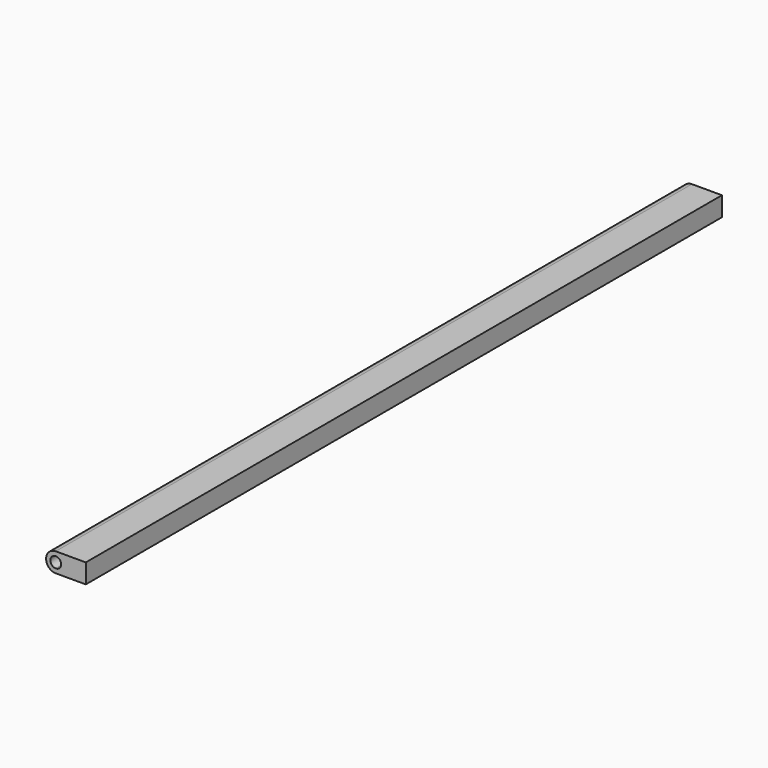
from build123d import *

# Parameters (mm, degrees)
F1_DEPTH = 2540


with BuildPart() as f1:
    # F0 (on Front) → F1 (new body, symmetric)
    with BuildSketch(Plane.XZ):
        with BuildLine():
            ThreePointArc((-33.9077054523, -4.3846159242), (-52.0580848188, -48.2035079531), (-95.8769768476, -66.3538873196))
            Line((-95.8769768476, -66.3538873196), (95.8769768476, -66.3538873196))
            Line((95.8769768476, -66.3538873196), (95.8769768476, 57.5846554711))
            Line((95.8769768476, 57.5846554711), (-95.8769768476, 57.5846554711))
            ThreePointArc((-95.8769768476, 57.5846554711), (-52.0580848188, 39.4342761046), (-33.9077054523, -4.3846159242))
        make_face()
        with BuildLine():
            ThreePointArc((-95.8769768476, 57.5846554711), (-157.846248243, -4.3846159242), (-95.8769768476, -66.3538873196))
            Line((-95.8769768476, -66.3538873196), (-95.8769768476, -38.9116128696))
            ThreePointArc((-95.8769768476, -38.9116128696), (-130.4039737931, -4.3846159242), (-95.8769768476, 30.1423810212))
            Line((-95.8769768476, 30.1423810212), (-95.8769768476, 57.5846554711))
        make_face()
        with BuildLine():
            Line((-95.8769768476, -38.9116128696), (-95.8769768476, -66.3538873196))
            ThreePointArc((-95.8769768476, -66.3538873196), (-52.0580848188, -48.2035079531), (-33.9077054523, -4.3846159242))
            ThreePointArc((-33.9077054523, -4.3846159242), (-52.0580848188, 39.4342761046), (-95.8769768476, 57.5846554711))
            Line((-95.8769768476, 57.5846554711), (-95.8769768476, 30.1423810212))
            ThreePointArc((-95.8769768476, 30.1423810212), (-71.4627031735, 20.0296577499), (-61.3499799022, -4.3846159242))
            ThreePointArc((-61.3499799022, -4.3846159242), (-71.4627031735, -28.7988895983), (-95.8769768476, -38.9116128696))
        make_face()
    extrude(amount=F1_DEPTH, both=True)


solid = f1.part
